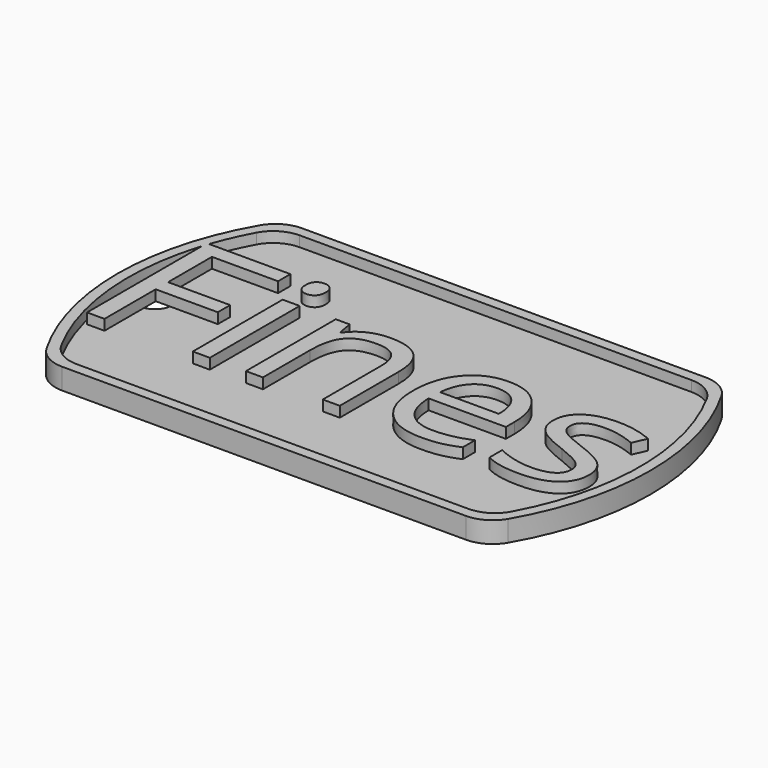
from build123d import *

# Parameters (mm, degrees)
F1_DEPTH     = 1
F3_DEPTH     = 1
F4_R         = 1.5875
F5_DEPTH     = 1
F6_TEXT_SIZE = 19.9990224145
F7_DEPTH     = 1


# Not quite as in the source:
# - a feature of the source that left no trace in its solid (it failed there, or was rolled back) is left out
# - Text() gives the source's letters only with a copy of the font that has no kerning and outlines rounded to 1/6400 em; it was checked with that copy


with BuildPart() as f1:
    # F0 (on Top) → F1 (new body)
    with BuildSketch(Plane.XY):
        with BuildLine():
            ThreePointArc((-19.2474145991, 14.2875), (-20.8349145991, 13.862130657), (-21.9970452561, 12.7))
            ThreePointArc((-21.9970452561, 12.7), (-25.4, 0), (-21.9970452561, -12.7))
            ThreePointArc((-21.9970452561, -12.7), (-20.8349145991, -13.862130657), (-19.2474145991, -14.2875))
            Line((-19.2474145991, -14.2875), (19.2474145991, -14.2875))
            ThreePointArc((19.2474145991, -14.2875), (20.8349145991, -13.862130657), (21.9970452561, -12.7))
            ThreePointArc((21.9970452561, -12.7), (25.4, 0), (21.9970452561, 12.7))
            ThreePointArc((21.9970452561, 12.7), (20.8349145991, 13.862130657), (19.2474145991, 14.2875))
            Line((19.2474145991, 14.2875), (-19.2474145991, 14.2875))
        make_face()
    extrude(amount=F1_DEPTH)

    # F2 (on face) → F3 (join)
    with BuildSketch(Plane.XY.offset(1)):
        with BuildLine():
            Line((19.2474145991, 14.2875), (-19.2474145991, 14.2875))
            ThreePointArc((-19.2474145991, 14.2875), (-20.8349145991, 13.862130657), (-21.9970452561, 12.7))
            ThreePointArc((-21.9970452561, 12.7), (-25.4, 0), (-21.9970452561, -12.7))
            ThreePointArc((-21.9970452561, -12.7), (-20.8349145991, -13.862130657), (-19.2474145991, -14.2875))
            Line((-19.2474145991, -14.2875), (19.2474145991, -14.2875))
            ThreePointArc((19.2474145991, -14.2875), (20.8349145991, -13.862130657), (21.9970452561, -12.7))
            ThreePointArc((21.9970452561, -12.7), (25.4, 0), (21.9970452561, 12.7))
            ThreePointArc((21.9970452561, 12.7), (20.8349145991, 13.862130657), (19.2474145991, 14.2875))
        make_face()
        with BuildLine():
            ThreePointArc((-21.4526124879, 11.6252061249), (-20.2856017842, 12.8404540819), (-18.6611352482, 13.2875))
            Line((-18.6611352482, 13.2875), (18.6611352482, 13.2875))
            ThreePointArc((18.6611352482, 13.2875), (20.2856017842, 12.8404540819), (21.4526124879, 11.6252061249))
            ThreePointArc((21.4526124879, 11.6252061249), (24.4, 0), (21.4526124879, -11.6252061249))
            ThreePointArc((21.4526124879, -11.6252061249), (20.2856017842, -12.8404540819), (18.6611352482, -13.2875))
            Line((18.6611352482, -13.2875), (-18.6611352482, -13.2875))
            ThreePointArc((-18.6611352482, -13.2875), (-20.2856017842, -12.8404540819), (-21.4526124879, -11.6252061249))
            ThreePointArc((-21.4526124879, -11.6252061249), (-24.4, 0), (-21.4526124879, 11.6252061249))
        make_face(mode=Mode.SUBTRACT)
    extrude(amount=F3_DEPTH)

    # F4 (on face) → F5 (cut)
    with BuildSketch(Plane.XY.offset(1)):
        with Locations((-21.821282804, 0)):
            Circle(F4_R)
    extrude(amount=-F5_DEPTH, mode=Mode.SUBTRACT)

    # F6 (on face) → F7 (join)
    with BuildSketch(Plane.XY.offset(1)):
        with Locations((-25.2211603203, -6.2974705367)):
            Text('Fines', F6_TEXT_SIZE, font='Open Sans', text_align=(TextAlign.LEFT, TextAlign.BOTTOM))
    extrude(amount=F7_DEPTH)


solid = f1.part
